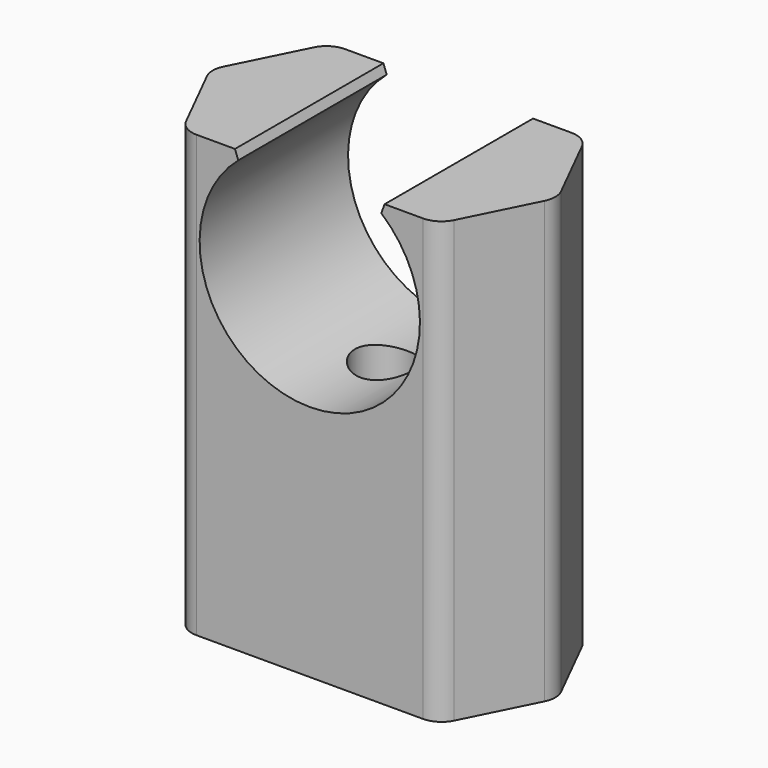
from build123d import *

# Parameters (mm, degrees)
F0_R        = 2.5
F1_DEPTH    = 20
F2_DEPTH    = 18
F4_DEPTH    = 12.5
F5_R        = 2
F6_T1_DEPTH = 22.7492112937


# Not quite as in the source:
# - a fillet or chamfer that OpenCascade refuses, or shapes differently, is made with other operations: its cross-section is extruded or revolved along the edge and cut away or added


with BuildPart() as f1:
    # F0 (on Top) → F1 (new body)
    with BuildSketch(Plane.XY):
        Polygon((11, 8), (-11, 8), (-15, 0), (-11, -8), (11, -8), (15, 0), align=None)
        Circle(F0_R, mode=Mode.SUBTRACT)
    extrude(amount=F1_DEPTH)

    # F2 (add): a face of the model
    f2_faces = [f1.faces().sort_by_distance(p)[0] for p in [
        (0, 7.66, 20),
    ]]
    extrude(f2_faces, amount=F2_DEPTH)

    # F3 (on Front) → F4 (cut, symmetric)
    with BuildSketch(Plane.XZ):
        with BuildLine():
            Line((5, 38.0777472107), (-5, 38.0777472107))
            ThreePointArc((-5, 38.0777472107), (0, 20.5), (5, 38.0777472107))
        make_face()
    extrude(amount=F4_DEPTH, both=True, mode=Mode.SUBTRACT)

    # F5
    f5_edges = [f1.edges().sort_by_distance(p)[0] for p in [
        (11, -8, 19),
        (15, 0, 19),
        (11, 8, 19),
        (-11, -8, 19),
        (-15, 0, 19),
        (-11, 8, 19),
    ]]
    fillet(f5_edges, radius=F5_R)

    # F6: chamfer of 1.5 on 2 edges, made by hand

    # F6_s2 → F6_t1 (cut)
    with BuildSketch(Plane.XZ.offset(-11.3746056469)):
        with BuildLine():
            Line((-6.4721431849, 38.0562963897), (-6.1455853598, 37.1704776118))
            Line((-6.1455853598, 37.1704776118), (-6.1261127101, 37.1476562202))
            ThreePointArc((-6.1261127101, 37.1476562202), (-5.6470472065, 37.6020890449), (-5.107295987, 37.9747368421))
            Line((-5.107295987, 37.9747368421), (-5.123475383, 38.03))
            ThreePointArc((-5.123475383, 38.03), (-5.7978092839, 38.03), (-6.4721431849, 38.0862963897))
            Line((-6.4721431849, 38.0862963897), (-6.4721431849, 38.0562963897))
        make_face()
        with BuildLine():
            Line((6.4721431849, 38.0562963897), (6.1455853598, 37.1704776118))
            Line((6.1455853598, 37.1704776118), (6.1261127101, 37.1476562202))
            ThreePointArc((6.1261127101, 37.1476562202), (5.6470472065, 37.6020890449), (5.107295987, 37.9747368421))
            Line((5.107295987, 37.9747368421), (5.123475383, 38.03))
            ThreePointArc((5.123475383, 38.03), (5.7978092839, 38.03), (6.4721431849, 38.0862963897))
            Line((6.4721431849, 38.0862963897), (6.4721431849, 38.0562963897))
        make_face()
    extrude(amount=F6_T1_DEPTH, mode=Mode.SUBTRACT)


solid = f1.part
